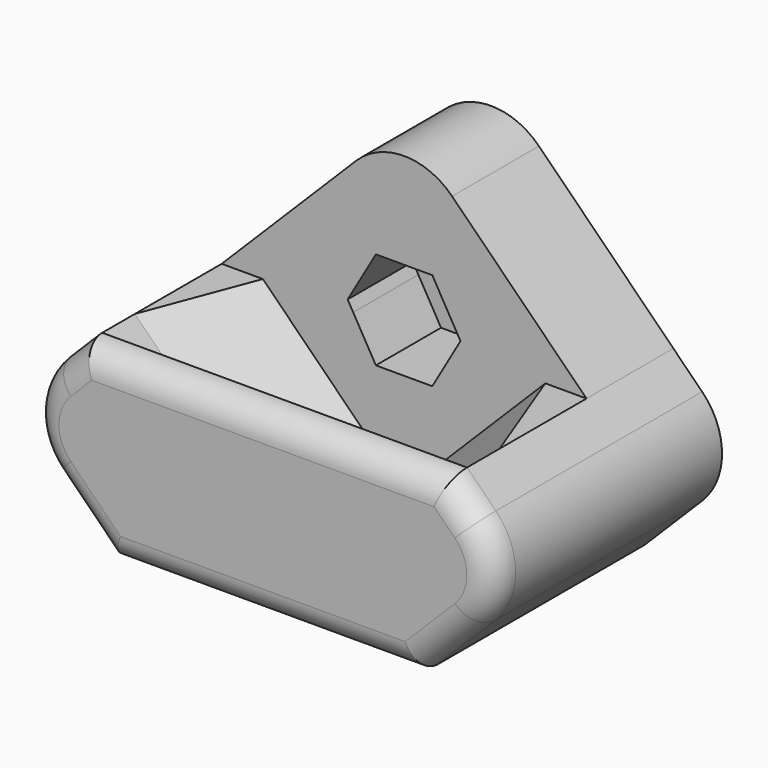
from build123d import *

# Parameters (mm, degrees)
F1_DEPTH = 8
F2_DEPTH = 6
F3_DEPTH = 13
F6_DEPTH = 8
F6_TAPER = 15
F7_DEPTH = 3
F8_R     = 5
F9_R     = 1.99999


# Not quite as in the source:
# - a fillet or chamfer is up to 0.001 mm smaller than in the source, because OpenCascade refuses the exact size


with BuildPart() as f1:
    # F0 (on Front) → F1 (new body)
    with BuildSketch(Plane.XZ):
        Polygon((-13.4350288425, 13.4350288425), (0, 0), (13.4350288425, 13.4350288425), (3.7486736477, 13.4350288425), (2.0784609691, 10.5421356237), (-2.0784609691, 10.5421356237), (-3.7486736477, 13.4350288425), align=None)
        Polygon((3.7486736477, 13.4350288425), (13.4350288425, 13.4350288425), (0, 26.8700576851), (-13.4350288425, 13.4350288425), (-3.7486736477, 13.4350288425), (-4.1569219382, 14.1421356237), (-2.0784609691, 17.7421356237), (2.0784609691, 17.7421356237), (4.1569219382, 14.1421356237), align=None)
        Polygon((-11.313708499, 0), (0, 0), (-13.4350288425, 13.4350288425), (-19.091883092, 7.7781745931), align=None)
        Polygon((13.4350288425, 13.4350288425), (0, 0), (11.313708499, 0), (19.091883092, 7.7781745931), align=None)
        with BuildLine():
            Line((1.8708286934, 13.4350288425), (3.7486736477, 13.4350288425))
            Line((3.7486736477, 13.4350288425), (4.1569219382, 14.1421356237))
            Line((4.1569219382, 14.1421356237), (2.0784609691, 17.7421356237))
            Line((2.0784609691, 17.7421356237), (-2.0784609691, 17.7421356237))
            Line((-2.0784609691, 17.7421356237), (-4.1569219382, 14.1421356237))
            Line((-4.1569219382, 14.1421356237), (-3.7486736477, 13.4350288425))
            Line((-3.7486736477, 13.4350288425), (-1.8708286934, 13.4350288425))
            ThreePointArc((-1.8708286934, 13.4350288425), (-0.3594040993, 16.109577794), (2, 14.1421356237))
            ThreePointArc((2, 14.1421356237), (1.9674421703, 13.7827315244), (1.8708286934, 13.4350288425))
        make_face()
        with BuildLine():
            Line((2.0784609691, 10.5421356237), (3.7486736477, 13.4350288425))
            Line((3.7486736477, 13.4350288425), (1.8708286934, 13.4350288425))
            ThreePointArc((1.8708286934, 13.4350288425), (0, 12.1421356237), (-1.8708286934, 13.4350288425))
            Line((-1.8708286934, 13.4350288425), (-3.7486736477, 13.4350288425))
            Line((-3.7486736477, 13.4350288425), (-2.0784609691, 10.5421356237))
            Line((-2.0784609691, 10.5421356237), (2.0784609691, 10.5421356237))
        make_face()
    extrude(amount=-F1_DEPTH)

    # F0 (on Front) → F2 (cut)
    with BuildSketch(Plane.XZ):
        with BuildLine():
            Line((1.8708286934, 13.4350288425), (3.7486736477, 13.4350288425))
            Line((3.7486736477, 13.4350288425), (4.1569219382, 14.1421356237))
            Line((4.1569219382, 14.1421356237), (2.0784609691, 17.7421356237))
            Line((2.0784609691, 17.7421356237), (-2.0784609691, 17.7421356237))
            Line((-2.0784609691, 17.7421356237), (-4.1569219382, 14.1421356237))
            Line((-4.1569219382, 14.1421356237), (-3.7486736477, 13.4350288425))
            Line((-3.7486736477, 13.4350288425), (-1.8708286934, 13.4350288425))
            ThreePointArc((-1.8708286934, 13.4350288425), (-0.3594040993, 16.109577794), (2, 14.1421356237))
            ThreePointArc((2, 14.1421356237), (1.9674421703, 13.7827315244), (1.8708286934, 13.4350288425))
        make_face()
        with BuildLine():
            Line((2.0784609691, 10.5421356237), (3.7486736477, 13.4350288425))
            Line((3.7486736477, 13.4350288425), (1.8708286934, 13.4350288425))
            ThreePointArc((1.8708286934, 13.4350288425), (0, 12.1421356237), (-1.8708286934, 13.4350288425))
            Line((-1.8708286934, 13.4350288425), (-3.7486736477, 13.4350288425))
            Line((-3.7486736477, 13.4350288425), (-2.0784609691, 10.5421356237))
            Line((-2.0784609691, 10.5421356237), (2.0784609691, 10.5421356237))
        make_face()
    extrude(amount=-F2_DEPTH, mode=Mode.SUBTRACT)

    # F0 (on Front) → F3 (join)
    with BuildSketch(Plane.XZ):
        Polygon((-11.313708499, 0), (0, 0), (-13.4350288425, 13.4350288425), (-19.091883092, 7.7781745931), align=None)
        Polygon((-13.4350288425, 13.4350288425), (0, 0), (13.4350288425, 13.4350288425), (3.7486736477, 13.4350288425), (2.0784609691, 10.5421356237), (-2.0784609691, 10.5421356237), (-3.7486736477, 13.4350288425), align=None)
        Polygon((13.4350288425, 13.4350288425), (0, 0), (11.313708499, 0), (19.091883092, 7.7781745931), align=None)
        with BuildLine():
            ThreePointArc((-1.8708286934, 13.4350288425), (0, 12.1421356237), (1.8708286934, 13.4350288425))
            Line((1.8708286934, 13.4350288425), (0, 13.4350288425))
            Line((0, 13.4350288425), (-1.8708286934, 13.4350288425))
        make_face()
        with BuildLine():
            Line((2.0784609691, 10.5421356237), (3.7486736477, 13.4350288425))
            Line((3.7486736477, 13.4350288425), (1.8708286934, 13.4350288425))
            ThreePointArc((1.8708286934, 13.4350288425), (0, 12.1421356237), (-1.8708286934, 13.4350288425))
            Line((-1.8708286934, 13.4350288425), (-3.7486736477, 13.4350288425))
            Line((-3.7486736477, 13.4350288425), (-2.0784609691, 10.5421356237))
            Line((-2.0784609691, 10.5421356237), (2.0784609691, 10.5421356237))
        make_face()
    extrude(amount=F3_DEPTH)

    # F5 (on offset) → F6 (cut)
    with BuildSketch(Plane.XZ.offset(8)):
        with BuildLine():
            Line((0, 26.8700576851), (-13.4350288425, 13.4350288425))
            Line((-13.4350288425, 13.4350288425), (-3.5355339059, 3.5355339059))
            ThreePointArc((-3.5355339059, 3.5355339059), (0, 2.0710678119), (3.5355339059, 3.5355339059))
            Line((3.5355339059, 3.5355339059), (13.4350288425, 13.4350288425))
            Line((13.4350288425, 13.4350288425), (0, 26.8700576851))
        make_face()
    extrude(amount=-F6_DEPTH, taper=F6_TAPER, mode=Mode.SUBTRACT)

    # F5 (on offset) → F7 (cut)
    with BuildSketch(Plane.XZ.offset(8)):
        with BuildLine():
            Line((0, 26.8700576851), (-13.4350288425, 13.4350288425))
            Line((-13.4350288425, 13.4350288425), (-3.5355339059, 3.5355339059))
            ThreePointArc((-3.5355339059, 3.5355339059), (0, 2.0710678119), (3.5355339059, 3.5355339059))
            Line((3.5355339059, 3.5355339059), (13.4350288425, 13.4350288425))
            Line((13.4350288425, 13.4350288425), (0, 26.8700576851))
        make_face()
    extrude(amount=F7_DEPTH, mode=Mode.SUBTRACT)

    # F8
    f8_edges = [f1.edges().sort_by_distance(p)[0] for p in [
        (-19.091883, -2.5, 7.778175),
        (0, 4, 26.870058),
        (19.091883, -2.5, 7.778175),
    ]]
    fillet(f8_edges, radius=F8_R)

    # F9 (radius 2 in the source; OpenCascade refuses exactly that, so slightly less here)
    f9_edges = [f1.edges().sort_by_distance(p)[0] for p in [
        (-14.495689, -13, 12.374369),
        (-17.020815, -13, 7.778175),
        (0, -13, 13.435029),
        (-13.435029, -13, 2.12132),
        (14.495689, -13, 12.374369),
        (0, -13, 0),
        (17.020815, -13, 7.778175),
        (13.435029, -13, 2.12132),
    ]]
    fillet(f9_edges, radius=F9_R)


solid = f1.part
